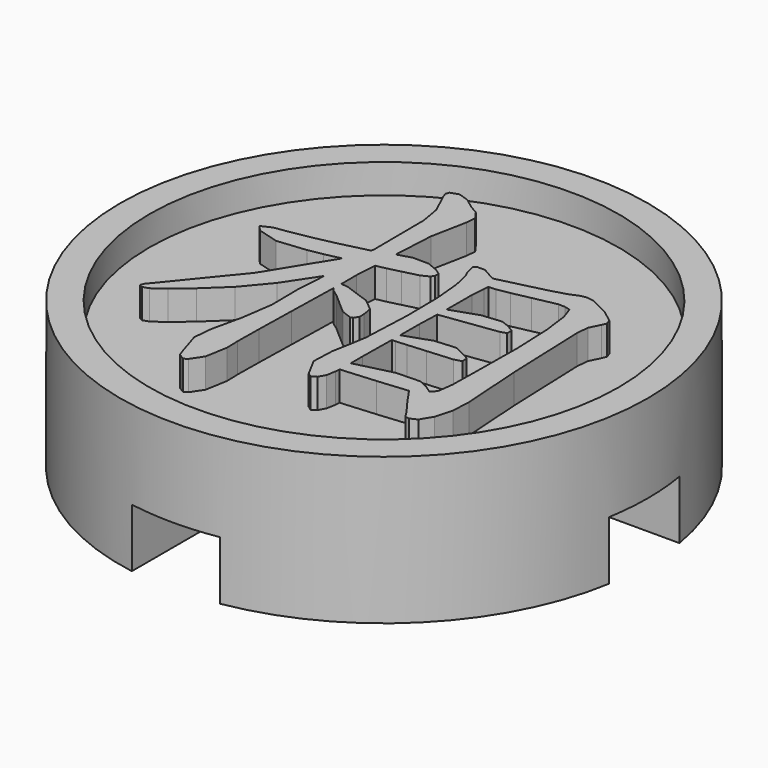
from build123d import *

# Parameters (mm, degrees)
F0_R     = 9
F1_DEPTH = 4
F3_W     = 3
F3_H     = 3
F4_DEPTH = 2
F2_R     = 9
F2_R_2   = 8
F5_DEPTH = 1
F7_DEPTH = 1


# Not quite as in the source:
# - a feature names something its author has since deleted; it is built from what else it names


with BuildPart() as f1:
    # F0 (on Top) → F1 (new body)
    with BuildSketch(Plane.XY):
        with Locations((-31.3306450844, 19.7580661625)):
            Circle(F0_R)
    extrude(amount=F1_DEPTH)

    # F3 (on face) → F4 (cut)
    with BuildSketch(Plane(origin=(0, 0, 0), x_dir=(1, 0, 0), z_dir=(0, 0, -1))):
        with BuildLine():
            ThreePointArc((-32.8306450844, -28.6321858371), (-32.0832814269, -28.7265408676), (-31.3306450844, -28.7580661625))
            ThreePointArc((-31.3306450844, -28.7580661625), (-30.5780087419, -28.7265408676), (-29.8306450844, -28.6321858371))
            Line((-29.8306450844, -28.6321858371), (-29.8306450844, -21.2580661625))
            Line((-29.8306450844, -21.2580661625), (-32.8306450844, -21.2580661625))
            Line((-32.8306450844, -21.2580661625), (-32.8306450844, -28.6321858371))
        make_face()
        with BuildLine():
            ThreePointArc((-40.204764759, -18.2580661625), (-40.2991197895, -19.0054298199), (-40.3306450844, -19.7580661625))
            ThreePointArc((-40.3306450844, -19.7580661625), (-40.2991197895, -20.510702505), (-40.204764759, -21.2580661625))
            Line((-40.204764759, -21.2580661625), (-32.8306450844, -21.2580661625))
            Line((-32.8306450844, -21.2580661625), (-32.8306450844, -18.2580661625))
            Line((-32.8306450844, -18.2580661625), (-40.204764759, -18.2580661625))
        make_face()
        with Locations((-31.3306450844, -19.7580661625)):
            Rectangle(F3_W, F3_H)
        with BuildLine():
            Line((-29.8306450844, -18.2580661625), (-29.8306450844, -21.2580661625))
            Line((-29.8306450844, -21.2580661625), (-22.4565254097, -21.2580661625))
            ThreePointArc((-22.4565254097, -21.2580661625), (-22.3621703793, -20.510702505), (-22.3306450844, -19.7580661625))
            ThreePointArc((-22.3306450844, -19.7580661625), (-22.3621703793, -19.0054298199), (-22.4565254097, -18.2580661625))
            Line((-22.4565254097, -18.2580661625), (-29.8306450844, -18.2580661625))
        make_face()
        with BuildLine():
            Line((-32.8306450844, -10.8839464878), (-32.8306450844, -18.2580661625))
            Line((-32.8306450844, -18.2580661625), (-29.8306450844, -18.2580661625))
            Line((-29.8306450844, -18.2580661625), (-29.8306450844, -10.8839464878))
            ThreePointArc((-29.8306450844, -10.8839464878), (-30.5780087419, -10.7895914574), (-31.3306450844, -10.7580661625))
            ThreePointArc((-31.3306450844, -10.7580661625), (-32.0832814269, -10.7895914574), (-32.8306450844, -10.8839464878))
        make_face()
    extrude(amount=-F4_DEPTH, mode=Mode.SUBTRACT)

    # F2 (on face) → F5 (join)
    with BuildSketch(Plane.XY.offset(4)):
        with Locations((-31.3306450844, 19.7580661625)):
            Circle(F2_R)
        with Locations((-31.3306450844, 19.7580661625)):
            Circle(F2_R_2, mode=Mode.SUBTRACT)
    extrude(amount=F5_DEPTH)

    # F6 (on face) → F7 (join)
    with BuildSketch(Plane.XY.offset(4)):
        Polygon((-32.8760972108, 17.7406868733), (-32.8363311232, 19.4874965841), (-32.7320557473, 19.367339138), (-32.5323725379, 19.2259714021), (-31.7937120117, 18.5827187093), (-31.4367533491, 18.4484232072), (-31.357221174, 18.4793473995), (-31.2600244437, 18.6251264653), (-31.2662246705, 18.8310099015), (-31.3165766676, 19.1446759774), (-31.7097685067, 19.4707104478), (-32.6030564059, 19.7879030229), (-32.7470978694, 19.79675133), (-32.8221930673, 19.8020410789), (-32.8257195665, 20.4594382394), (-32.7797853112, 21.1875000325), (-32.4431392841, 21.2572605989), (-32.0128486731, 21.3642097024), (-31.4915359115, 21.4958443005), (-31.2317483318, 21.625747708), (-31.1699063592, 21.7309015029), (-31.1646166104, 21.8837592145), (-31.3731224796, 22.022446811), (-31.7406862871, 22.173573332), (-32.2823373316, 22.1762021769), (-32.7515091993, 22.0357192717), (-32.6746251046, 23.4326617891), (-32.4369647045, 24.6475728288), (-32.4033731965, 24.985090863), (-32.6030564059, 25.2625301742), (-32.8902352667, 25.4294938826), (-33.2321710427, 25.6866718529), (-33.5873664558, 25.8059316446), (-33.8612664441, 25.7149479648), (-33.9045590309, 25.5947264005), (-33.8471283882, 25.4286603465), (-33.516676176, 24.7182310495), (-33.3982883913, 24.043194981), (-33.3841503354, 21.8837592145), (-33.4018148906, 21.8325287985), (-33.3982883913, 21.8024573779), (-34.3693195687, 21.5647713307), (-35.1689628841, 21.394281123), (-35.8015976083, 21.280279021), (-36.2716607186, 21.2122496452), (-36.615369362, 21.0514412809), (-36.4377703731, 20.8588303054), (-35.7326834018, 20.660897522), (-34.7660507307, 20.7598318546), (-34.26506984, 20.8490843439), (-33.7269709421, 20.9683441357), (-35.0205229143, 18.8698719229), (-36.9290373614, 16.5293023329), (-36.9767502546, 16.4117929671), (-36.8618857633, 16.3525734275), (-36.6568961344, 16.4214940459), (-36.2548745824, 16.7077688405), (-35.6734830977, 17.2034728061), (-34.9321616675, 17.9006039951), (-34.1987908902, 18.7779905887), (-33.4654265246, 19.8833365036), (-33.5308142319, 18.8195199258), (-33.5184458374, 17.7062105346), (-33.6765997096, 16.6309039812), (-33.9036742002, 15.6103799903), (-33.9646569894, 14.9591894683), (-33.7128328861, 14.1613222262), (-33.6368336221, 13.9421958237), (-33.5078342807, 13.8573726174), (-33.4265645033, 13.8070090791), (-33.2993284115, 13.885647447), (-33.0351359137, 14.2841392939), (-32.903488492, 15.0378239891), (-32.9167417172, 15.5034693576), (-32.9052517416, 16.4082408206), align=None)
        Polygon((-29.7933085363, 15.7623528711), (-29.7827290386, 15.9284702197), (-28.5978253014, 16.0212427964), (-27.5666769301, 16.1193243574), (-27.2115263998, 15.6050774178), (-26.8527852521, 15.119113002), (-26.718457691, 14.8999891642), (-26.5664976337, 14.8717130523), (-26.3376598936, 14.9821630078), (-26.0999738463, 15.3806510076), (-25.9417943268, 15.9558550891), (-25.9090940614, 16.5964597016), (-26.0487434304, 18.686968438), (-26.1565260701, 21.5267492573), (-26.1149774975, 21.9367849391), (-25.9373701733, 22.2937307781), (-25.873764951, 22.4465884896), (-25.9373701733, 22.618874006), (-26.3279139321, 22.9157411219), (-26.9622990823, 23.2373578506), (-27.2317877407, 23.2833305768), (-27.4429929848, 23.2373578506), (-27.754863752, 23.1075185612), (-28.2576784223, 22.9634450386), (-28.961888257, 22.7885306774), (-29.878136872, 22.5658482814), (-30.0972286507, 22.6886986905), (-30.3411341603, 22.827386287), (-30.6309354542, 22.827386287), (-30.6980928229, 22.7408267607), (-30.6592051543, 22.5941243933), (-30.6194454785, 22.4077328801), (-30.5496464413, 22.2831512804), (-30.4100611904, 21.6999965461), (-30.3243352003, 20.7651536625), (-30.3101650853, 19.4662991179), (-30.383516269, 17.7910388703), (-30.4780905662, 17.2237854416), (-30.5885020508, 16.6247294017), (-30.6176758171, 15.8683850849), (-30.2740024388, 15.2286781268), (-30.1308265705, 15.1279484855), (-29.9735447054, 15.2286781268), (-29.8480654514, 15.4601703591), align=None)
        Polygon((-27.3688082649, 16.5973381205), (-27.6621488817, 16.734275291), (-28.4926715066, 16.7086729067), (-29.7685589236, 16.3914546843), (-29.7720854228, 16.8906659136), (-29.7544529267, 18.119721421), (-29.6351290168, 18.1223887368), (-29.2604865636, 18.1515432676), (-28.6375785653, 18.2010168457), (-27.7717268301, 18.2681742145), (-27.523397167, 18.3415061628), (-27.5384008182, 18.5438374524), (-28.1145025541, 18.8442695385), (-28.8478861551, 18.7877173147), (-29.7544529267, 18.4731471727), (-29.7491311188, 19.2913398739), (-29.7261768148, 20.0211777403), (-27.800002942, 20.2827285695), (-27.6046990035, 20.349860291), (-27.594953042, 20.5300964601), (-27.8309078988, 20.6732723284), (-28.1145025541, 20.7881079665), (-28.7754326257, 20.7209762451), (-29.7120066998, 20.4064125148), (-29.7093778549, 21.4825718398), (-29.6731510902, 21.9544174351), (-29.6589809752, 22.1170211082), (-29.4142419295, 22.1293959145), (-28.9768919083, 22.2089024423), (-28.3601392541, 22.3388058499), (-27.5808470451, 22.4987165599), (-27.3564334586, 22.496087715), (-27.1567053665, 22.4456908353), (-27.0091694628, 22.0215491566), (-26.9004891688, 21.1521709222), (-26.8474634442, 19.8303171908), (-26.8668912489, 18.0490311413), (-26.8827925545, 17.127473542), (-26.9481930855, 16.6247294017), (-27.0348167299, 16.4789246886), (-27.1284292546, 16.4338688522), align=None, mode=Mode.SUBTRACT)
    extrude(amount=F7_DEPTH)


solid = f1.part
